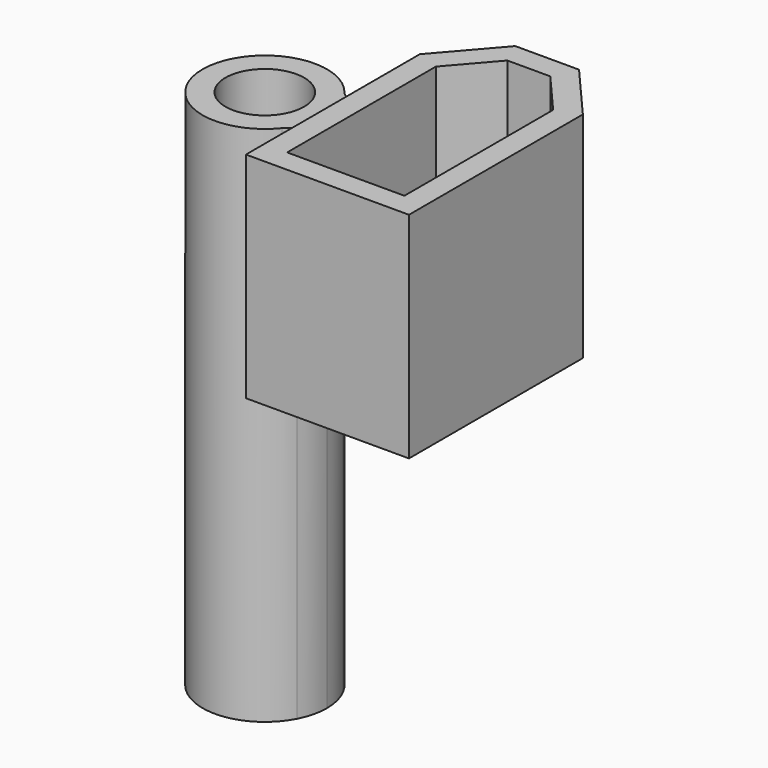
from build123d import *

# Parameters (mm, degrees)
F1_DEPTH      = 15
F2_DEPTH      = 13
F0_R          = 2.75
F3_DEPTH      = 13
F3_DEPTH_BACK = 23.5
F4_T1_DEPTH   = 13


# Not quite as in the source:
# - a fillet or chamfer that OpenCascade refuses, or shapes differently, is made with other operations: its cross-section is extruded or revolved along the edge and cut away or added


with BuildPart() as f1:
    # F0 (on Top) → F1 (new body)
    with BuildSketch(Plane.XY):
        Polygon((2.2306062124, 9.8), (0, 9.8), (-2.2306062124, 9.8), (-5.7, 5.796853322), (-5.7, 2), (-5.7, -2), (-5.7, -9.4), (0, -9.4), (5.7, -9.4), (5.7, 5.796853322), align=None)
        Polygon((-1.5, 8.2), (0, 8.2), (1.5, 8.2), (4.1, 5.2), (4.1, -7.8), (0, -7.8), (-4.1, -7.8), (-4.1, 5.2), align=None, mode=Mode.SUBTRACT)
    extrude(amount=F1_DEPTH)

    # F0 (on Top) → F2 (join)
    with BuildSketch(Plane.XY):
        with BuildLine():
            Line((-5.7, -2), (-5.7, 2))
            Line((-5.7, 2), (-8.0370348177, 2))
            ThreePointArc((-8.0370348177, 2), (-7.6735121825, 1.0292233618), (-7.55, 0))
            ThreePointArc((-7.55, 0), (-7.6735121825, -1.0292233618), (-8.0370348177, -2))
            Line((-8.0370348177, -2), (-5.7, -2))
        make_face()
        with BuildLine():
            ThreePointArc((-7.55, 0), (-7.6735121825, 1.0292233618), (-8.0370348177, 2))
            Line((-8.0370348177, 2), (-8.4, 2))
            Line((-8.4, 2), (-8.4, -2))
            Line((-8.4, -2), (-8.0370348177, -2))
            ThreePointArc((-8.0370348177, -2), (-7.6735121825, -1.0292233618), (-7.55, 0))
        make_face()
    extrude(amount=F2_DEPTH)

    # F0 (on Top) → F3 (join, two sides)
    with BuildSketch(Plane.XY) as f3_sk:
        with BuildLine():
            Line((-8.4, 2), (-8.0370348177, 2))
            ThreePointArc((-8.0370348177, 2), (-16.25, 0), (-8.0370348177, -2))
            Line((-8.0370348177, -2), (-8.4, -2))
            Line((-8.4, -2), (-8.4, 2))
        make_face()
        with Locations((-11.9, 0)):
            Circle(F0_R, mode=Mode.SUBTRACT)
        with BuildLine():
            ThreePointArc((-7.55, 0), (-7.6735121825, 1.0292233618), (-8.0370348177, 2))
            Line((-8.0370348177, 2), (-8.4, 2))
            Line((-8.4, 2), (-8.4, -2))
            Line((-8.4, -2), (-8.0370348177, -2))
            ThreePointArc((-8.0370348177, -2), (-7.6735121825, -1.0292233618), (-7.55, 0))
        make_face()
    extrude(amount=F3_DEPTH)
    extrude(f3_sk.sketch, amount=-F3_DEPTH_BACK)

    # F4: fillet of radius 2 on 4 edges, made by hand

    # F4_s2 → F4_t1 (join)
    with BuildSketch(Plane.XY):
        with BuildLine():
            ThreePointArc((-5.7, -4), (-6.2857864376, -2.5857864376), (-7.7, -2))
            Line((-7.7, -2), (-5.7, -2))
            Line((-5.7, -2), (-5.7, -4))
        make_face()
        with BuildLine():
            ThreePointArc((-5.7, 4), (-6.2857864376, 2.5857864376), (-7.7, 2))
            Line((-7.7, 2), (-5.7, 2))
            Line((-5.7, 2), (-5.7, 4))
        make_face()
        with BuildLine():
            ThreePointArc((-6.9682153332, -2), (-7.8285393886, -2.1944966021), (-8.5215333385, -2.7401574803))
            ThreePointArc((-8.5215333385, -2.7401574803), (-8.2604200708, -2.382426901), (-8.0370348177, -2))
            Line((-8.0370348177, -2), (-6.9682153332, -2))
        make_face()
        with BuildLine():
            ThreePointArc((-6.9682153332, 2), (-7.8285393886, 2.1944966021), (-8.5215333385, 2.7401574803))
            ThreePointArc((-8.5215333385, 2.7401574803), (-8.2604200708, 2.382426901), (-8.0370348177, 2))
            Line((-8.0370348177, 2), (-6.9682153332, 2))
        make_face()
    extrude(amount=F4_T1_DEPTH)


solid = f1.part
